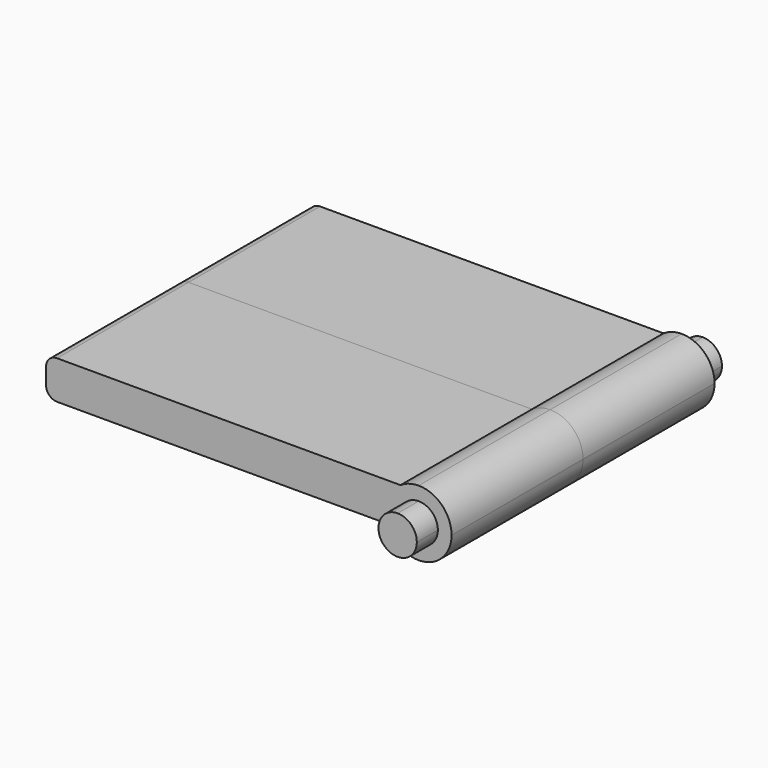
from build123d import *

# Parameters (mm, degrees)
F1_DEPTH = 2.4
F2_DEPTH = 15


with BuildPart() as f1:
    # F0 (on Front) → F1 (new body)
    with BuildSketch(Plane.XZ):
        with BuildLine():
            Line((0, -1), (0, 0))
            Line((0, 0), (0, 1.75))
            ThreePointArc((0, 1.75), (-1.5512092057, 0.8100925873), (-1.4361406616, -1))
            Line((-1.4361406616, -1), (0, -1))
        make_face()
        with BuildLine():
            Line((0, 1.75), (0, 0))
            Line((0, 0), (0, -1))
            Line((0, -1), (-1.4361406616, -1))
            ThreePointArc((-1.4361406616, -1), (0.5240485866, -1.6696925103), (1.75, 0))
            ThreePointArc((1.75, 0), (1.2374368671, 1.2374368671), (0, 1.75))
        make_face()
    extrude(amount=F1_DEPTH)

    # F0 (on Front) → F2 (join)
    with BuildSketch(Plane.XZ):
        with BuildLine():
            Line((0, -1), (0, 0))
            Line((0, 0), (0, 1.75))
            ThreePointArc((0, 1.75), (-1.5512092057, 0.8100925873), (-1.4361406616, -1))
            Line((-1.4361406616, -1), (0, -1))
        make_face()
        with BuildLine():
            Line((0, 1.75), (0, 0))
            Line((0, 0), (0, -1))
            Line((0, -1), (-1.4361406616, -1))
            ThreePointArc((-1.4361406616, -1), (0.5240485866, -1.6696925103), (1.75, 0))
            ThreePointArc((1.75, 0), (1.2374368671, 1.2374368671), (0, 1.75))
        make_face()
        with BuildLine():
            ThreePointArc((-1.4361406616, -1), (-1.5512092057, 0.8100925873), (0, 1.75))
            Line((0, 1.75), (0, 2.5))
            Line((0, 2.5), (-1.6583123952, 2.5))
            ThreePointArc((-1.6583123952, 2.5), (-2.8452078799, 0.951205614), (-2.8284271247, -1))
            Line((-2.8284271247, -1), (-1.4361406616, -1))
        make_face()
        with BuildLine():
            Line((0, 2.5), (0, 1.75))
            ThreePointArc((0, 1.75), (1.2374368671, 1.2374368671), (1.75, 0))
            ThreePointArc((1.75, 0), (0.5240485866, -1.6696925103), (-1.4361406616, -1))
            Line((-1.4361406616, -1), (-2.8284271247, -1))
            ThreePointArc((-2.8284271247, -1), (0.5073059362, -2.956795679), (3, 0))
            ThreePointArc((3, 0), (2.1213203436, 2.1213203436), (0, 3))
            Line((0, 3), (0, 2.5))
        make_face()
        with BuildLine():
            Line((-1.6583123952, 2.5), (0, 2.5))
            Line((0, 2.5), (0, 3))
            ThreePointArc((0, 3), (-0.8660254038, 2.8722813233), (-1.6583123952, 2.5))
        make_face()
        with BuildLine():
            ThreePointArc((-2.8284271247, -1), (-2.8452078799, 0.951205614), (-1.6583123952, 2.5))
            Line((-1.6583123952, 2.5), (-33, 2.5))
            ThreePointArc((-33, 2.5), (-33.7071067812, 2.2071067812), (-34, 1.5))
            Line((-34, 1.5), (-34, 0))
            ThreePointArc((-34, 0), (-33.7071067812, -0.7071067812), (-33, -1))
            Line((-33, -1), (-2.8284271247, -1))
        make_face()
    extrude(amount=-F2_DEPTH)


with BuildPart() as f3_1:
    # F3: instance of F1
    add(f1.part.mirror(Plane(origin=(-14.523910756, 15, 0.6034083125), x_dir=(1, 0, 0), z_dir=(0, 1, 0))))


solid = Compound([f1.part, f3_1.part])
